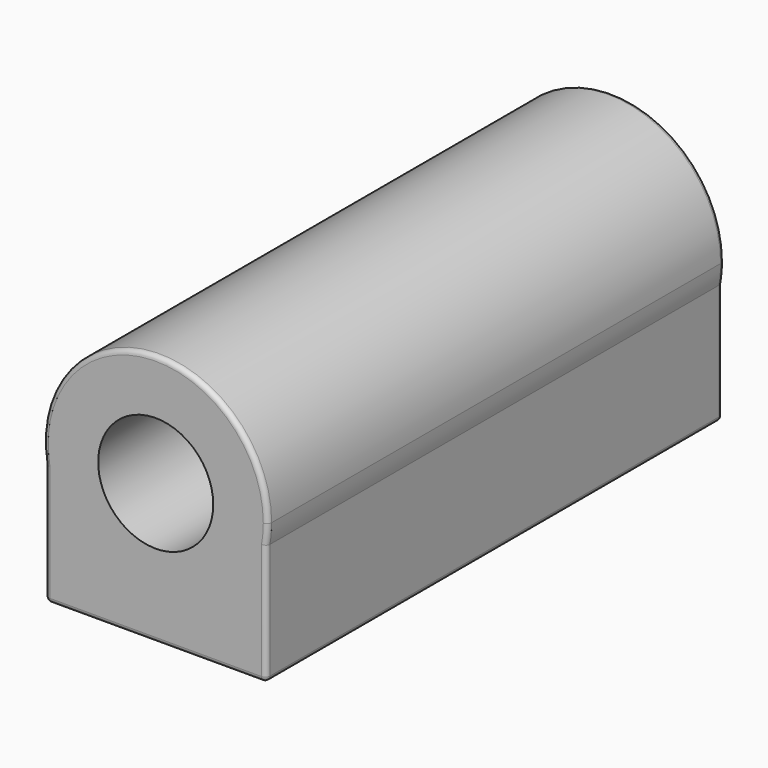
from build123d import *

# Parameters (mm, degrees)
F1_R     = 6.15
F2_DEPTH = 61
F3_DEPTH = 61.001
F4_DEPTH = 2
F5_R     = 0.5


# Not quite as in the source:
# - two fillets or chamfers of one size are made in one step


with BuildPart() as f2:
    # F1 (on face) → F2 (new body)
    with BuildSketch(Plane.XZ):
        Circle(F1_R)
    extrude(amount=F2_DEPTH)


with BuildPart() as f2b:
    # F0 (on Front) → F2, piece 2 (new body)
    with BuildSketch(Plane.XZ):
        with BuildLine():
            ThreePointArc((11.8124997243, -2.1130192291), (11.9530330187, -1.0606609515), (12, 0))
            ThreePointArc((12, 0), (-1.0606609515, 11.9530330187), (-11.8124997243, -2.1130192291))
            Line((-11.8124997243, -2.1130192291), (-11.8124997243, 1))
            Line((-11.8124997243, 1), (11.8124997243, 1))
            Line((11.8124997243, 1), (11.8124997243, -2.1130192291))
        make_face()
        with BuildLine():
            Line((-11.8124997243, 1), (-11.8124997243, -2.1130192291))
            ThreePointArc((-11.8124997243, -2.1130192291), (0, -12), (11.8124997243, -2.1130192291))
            Line((11.8124997243, -2.1130192291), (11.8124997243, 1))
            Line((11.8124997243, 1), (-11.8124997243, 1))
        make_face()
        with BuildLine():
            ThreePointArc((11.8124997243, -2.1130192291), (0, -12), (-11.8124997243, -2.1130192291))
            Line((-11.8124997243, -2.1130192291), (-11.8124997243, -13))
            Line((-11.8124997243, -13), (11.8124997243, -13))
            Line((11.8124997243, -13), (11.8124997243, -2.1130192291))
        make_face()
    extrude(amount=F2_DEPTH)


with BuildPart() as f3_tool:
    # F3 (cut, through all): a face of the model
    f3_faces = [f2.part.faces().sort_by_distance(p)[0] for p in [
        (0, -61, 0),
    ]]
    extrude(f3_faces, amount=-F3_DEPTH)


with BuildPart() as f2_1:
    add(f2.part)

    # F3: cut by f3_tool
    add(f3_tool.part, mode=Mode.SUBTRACT)


with BuildPart() as f2b_1:
    add(f2b.part)

    # F3: cut by f3_tool
    add(f3_tool.part, mode=Mode.SUBTRACT)

    # F4 (add): a face of the model
    f4_faces = [f2b_1.faces().sort_by_distance(p)[0] for p in [
        (0, -30.5, -13),
    ]]
    extrude(f4_faces, amount=F4_DEPTH)

    # F5
    f5_edges = [f2b_1.edges().sort_by_distance(p)[0] for p in [
        (0, -61, 12),
        (-11.8125, -61, -8.55651),
        (11.8125, -61, -8.55651),
        (11.8125, 0, -8.55651),
        (-11.8125, 0, -8.55651),
        (0, 0, 12),
        (-11.8125, -30.5, -15),
        (0, 0, -15),
        (11.8125, -30.5, -15),
        (0, -61, -15),
    ]]
    fillet(f5_edges, radius=F5_R)


solid = f2b_1.part
